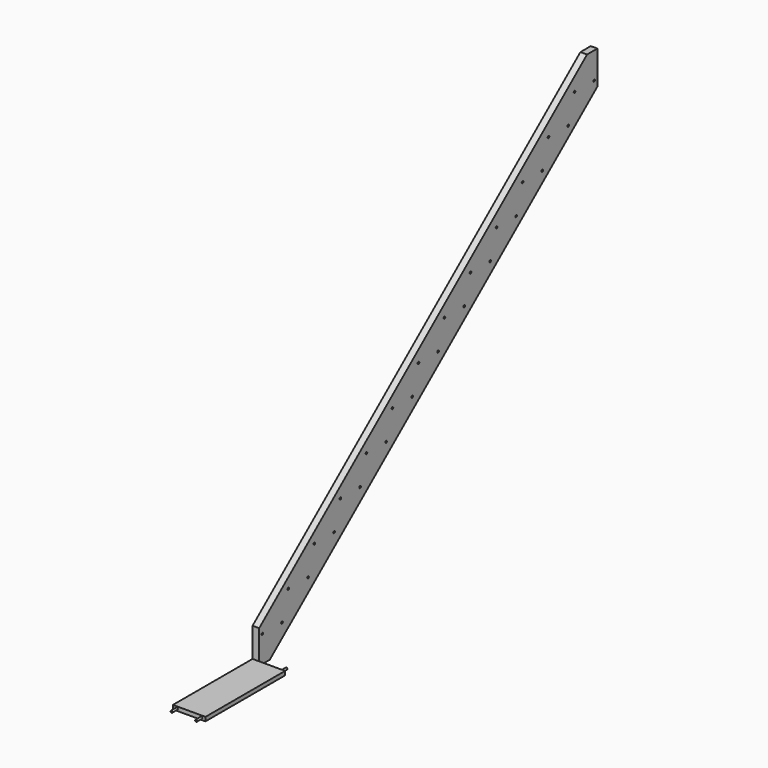
from build123d import *

# Parameters (mm, degrees)
F1_DEPTH      = 50
F2_D          = 15.5
F3_W          = 245
F3_H          = 30
F4_DEPTH      = 750
F5_R          = 7.5
F6_DEPTH      = 50
F6_DEPTH_BACK = 800


with BuildPart() as f1:
    # F0 (on Right) → F1 (new body)
    with BuildSketch(Plane.YZ):
        Polygon((0, 0), (100, 0), (3185, 2547.6726726727), (3185, 2800), (3087.8181818182, 2800), (0, 250), align=None)
    extrude(amount=F1_DEPTH)

    # F2 (through all)
    with Locations(Plane(origin=(0, 0, 0), x_dir=(0, 1, 0), z_dir=(-1, 0, 0))):
        with Locations((3400, -2800), (30, -200), (215, -200), (275, -400), (460, -400), (520, -600), (705, -600), (765, -800), (950, -800), (1010, -1000), (1195, -1000), (1255, -1200), (1440, -1200), (1500, -1400), (1685, -1400), (1745, -1600), (1930, -1600), (1990, -1800), (2175, -1800), (2235, -2000), (2420, -2000), (2480, -2200), (2665, -2200), (2725, -2400), (2910, -2400), (2970, -2600), (3155, -2600), (3215, -2800)):
            Hole(F2_D / 2)


with BuildPart() as f4:
    # F3 (on Front) → F4 (new body)
    with BuildSketch(Plane.XZ):
        with Locations((122.5, 15)):
            Rectangle(F3_W, F3_H)
    extrude(amount=F4_DEPTH)

    # F5 (on face) → F6 (join, two sides)
    with BuildSketch(Plane.XZ.offset(750)) as f6_sk:
        with Locations((30, 15)):
            Circle(F5_R)
        with Locations((215, 15)):
            Circle(F5_R)
    extrude(amount=F6_DEPTH)
    extrude(f6_sk.sketch, amount=-F6_DEPTH_BACK)


solid = Compound([f1.part, f4.part])
